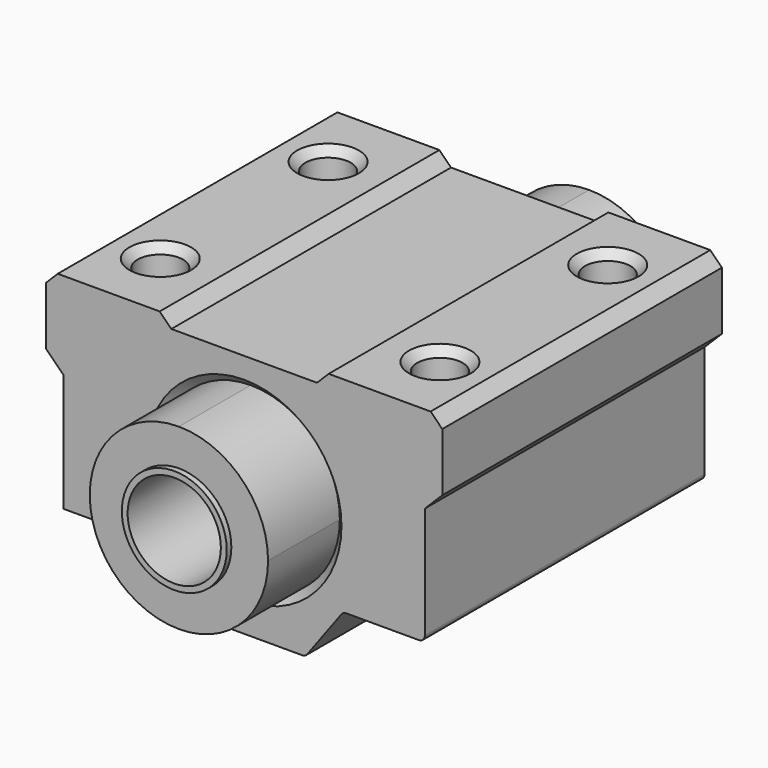
from build123d import *

# Parameters (mm, degrees)
F1_DEPTH       = 15
F2_SIZE        = 0.99999
F3_SIZE        = 1.49999
F4_R           = 0.5
F6_D           = 3.6
F6_CBORE_D     = 3.9
F6_CBORE_DEPTH = 6
F7_SIZE        = 0.7
F0_R           = 4.5
F8_DEPTH       = 22
F0_R_2         = 4
F9_DEPTH       = 22.5


# Not quite as in the source:
# - a fillet or chamfer is up to 0.001 mm smaller than in the source, because OpenCascade refuses the exact size


with BuildPart() as f1:
    # F0 (on Front) → F1 (new body, symmetric)
    with BuildSketch(Plane.XZ):
        with BuildLine():
            ThreePointArc((0, 7.65), (5.4093668761, 5.4093668761), (7.65, 0))
            ThreePointArc((7.65, 0), (5.4093668761, -5.4093668761), (0, -7.65))
            Line((0, -7.65), (0, -10.85))
            Line((0, -10.85), (5.25, -10.85))
            Line((5.25, -10.85), (8.5, -6.45))
            Line((8.5, -6.45), (15.5, -6.45))
            Line((15.5, -6.45), (15.5, 3.65))
            Line((15.5, 3.65), (17, 3.65))
            Line((17, 3.65), (17, 11.15))
            Line((17, 11.15), (7.25, 11.15))
            Line((7.25, 11.15), (7.25, 10.15))
            Line((7.25, 10.15), (0, 10.15))
            Line((0, 10.15), (0, 7.65))
        make_face()
        with BuildLine():
            ThreePointArc((0, -7.65), (-7.65, 0), (0, 7.65))
            Line((0, 7.65), (0, 10.15))
            Line((0, 10.15), (-7.25, 10.15))
            Line((-7.25, 10.15), (-7.25, 11.15))
            Line((-7.25, 11.15), (-17, 11.15))
            Line((-17, 11.15), (-17, 3.65))
            Line((-17, 3.65), (-15.5, 3.65))
            Line((-15.5, 3.65), (-15.5, -6.45))
            Line((-15.5, -6.45), (-8.5, -6.45))
            Line((-8.5, -6.45), (-5.25, -10.85))
            Line((-5.25, -10.85), (0, -10.85))
            Line((0, -10.85), (0, -7.65))
        make_face()
    extrude(amount=F1_DEPTH, both=True)

    # F2 (size 1 in the source; OpenCascade refuses exactly that, so slightly less here)
    f2_edges = [f1.edges().sort_by_distance(p)[0] for p in [
        (7.25, 0, 10.15),
        (17, 0, 11.15),
        (-7.25, 0, 10.15),
        (-17, 0, 11.15),
    ]]
    chamfer(f2_edges, length=F2_SIZE)

    # F3 (size 1.5 in the source; OpenCascade refuses exactly that, so slightly less here)
    f3_edges = [f1.edges().sort_by_distance(p)[0] for p in [
        (17, 0, 3.65),
        (-17, 0, 3.65),
    ]]
    chamfer(f3_edges, length=F3_SIZE)

    # F4
    f4_edges = [f1.edges().sort_by_distance(p)[0] for p in [
        (15.5, 0, -6.45),
        (8.5, 0, -6.45),
        (5.25, 0, -10.85),
        (-5.25, 0, -10.85),
        (-8.5, 0, -6.45),
    ]]
    fillet(f4_edges, radius=F4_R)

    # F6 (through all)
    with Locations(Plane.XY.offset(11.15)):
        with Locations((12, 9), (12, -9), (-12, 9), (-12, -9)):
            CounterBoreHole(F6_D / 2, F6_CBORE_D / 2, F6_CBORE_DEPTH)

    # F7
    f7_edges = [f1.edges().sort_by_distance(p)[0] for p in [
        (-7.65, -15, 0),
        (-7.65, 15, 0),
        (10.05, 9, 11.15),
        (10.05, -9, 11.15),
        (-13.95, 9, 11.15),
        (-13.95, -9, 11.15),
    ]]
    chamfer(f7_edges, length=F7_SIZE)


with BuildPart() as f8:
    # F0 (on Front) → F8 (new body, symmetric)
    with BuildSketch(Plane.XZ):
        with BuildLine():
            ThreePointArc((0, -7.65), (5.4093668761, -5.4093668761), (7.65, 0))
            ThreePointArc((7.65, 0), (5.4093668761, 5.4093668761), (0, 7.65))
            ThreePointArc((0, 7.65), (-7.65, 0), (0, -7.65))
        make_face()
        Circle(F0_R, mode=Mode.SUBTRACT)
    extrude(amount=F8_DEPTH, both=True)

    # F0 (on Front) → F9 (join, symmetric)
    with BuildSketch(Plane.XZ):
        Circle(F0_R)
        Circle(F0_R_2, mode=Mode.SUBTRACT)
    extrude(amount=F9_DEPTH, both=True)


solid = Compound([f1.part, f8.part])
